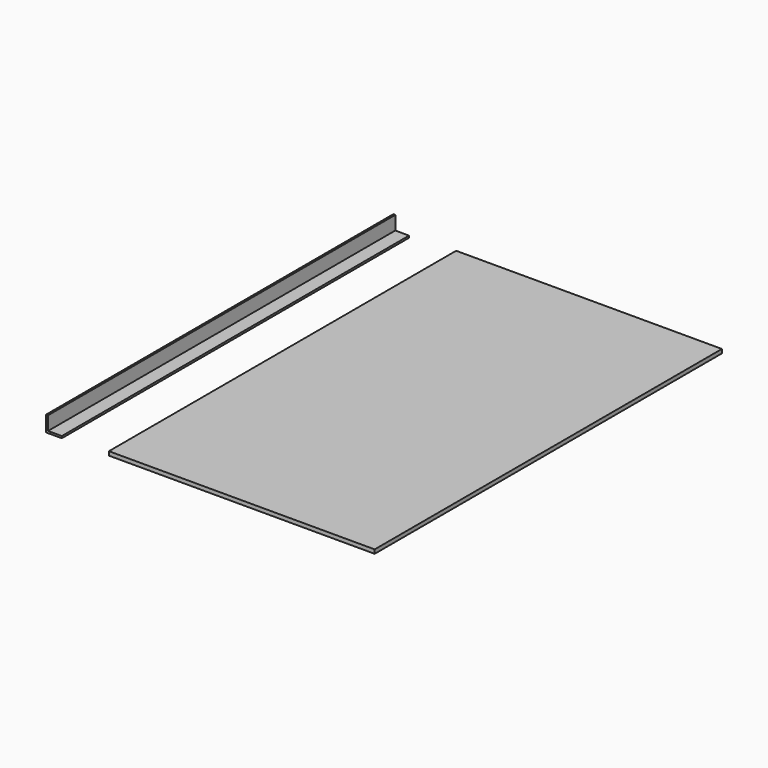
from build123d import *

# Parameters (mm, degrees)
F0_W     = 429.26
F0_H     = 701.04
F1_DEPTH = 6.35
F3_DEPTH = 701.04


# Not quite as in the source:
# - the program builds the solid bodies; features that only make, move or delete a surface that nothing else refers to are left out


with BuildPart() as f1:
    # F0 (on Top) → F1 (new body)
    with BuildSketch(Plane.XY):
        with Locations((214.63, -350.52)):
            Rectangle(F0_W, F0_H)
    extrude(amount=F1_DEPTH)


with BuildPart() as f3:
    # F2 (on Front) → F3 (new body)
    with BuildSketch(Plane.XZ):
        Polygon((-101.4562074584, 25.4), (-101.4562074584, 0), (-76.0562074584, 0), (-76.0562074584, 3.175), (-98.2812074584, 3.175), (-98.2812074584, 25.4), align=None)
    extrude(amount=F3_DEPTH)


solid = Compound([f1.part, f3.part])
